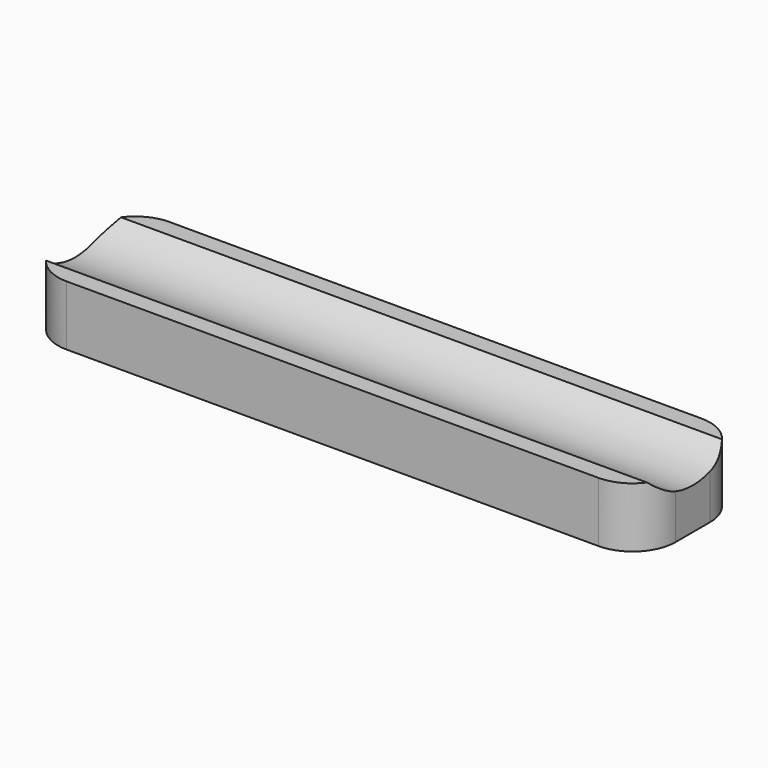
from build123d import *

# Parameters (mm, degrees)
F0_W      = 72
F0_H      = 15
F1_DEPTH  = 3.8
F3_DEPTH  = 72
F4_R      = 5
F5_W      = 36
F5_H      = 2
F6_DEPTH  = 1
F7_R      = 0.99999
F10_DEPTH = 4
F11_R     = 2
F12_R     = 1


# Not quite as in the source:
# - a fillet or chamfer is up to 0.001 mm smaller than in the source, because OpenCascade refuses the exact size
# - a pattern or mirror of a feature is missing from the dataset's text; its kind, count and spacing are read off the source's solid


with BuildPart() as f1:
    # F0 (on Top) → F1 (new body)
    with BuildSketch(Plane.XY):
        Rectangle(F0_W, F0_H)
    extrude(amount=F1_DEPTH)

    # F2 (on face) → F3 (join)
    with BuildSketch(Plane.YZ.offset(36)):
        with BuildLine():
            Line((7.5, 7), (5.4598534779, 7))
            ThreePointArc((5.4598534779, 7), (0, 4.8), (-5.4598534779, 7))
            Line((-5.4598534779, 7), (-7.5, 7))
            Line((-7.5, 7), (-7.5, 3.8))
            Line((-7.5, 3.8), (7.5, 3.8))
            Line((7.5, 3.8), (7.5, 7))
        make_face()
    extrude(amount=-F3_DEPTH)

    # F4
    f4_edges = [f1.edges().sort_by_distance(p)[0] for p in [
        (-36, -7.5, 3.5),
        (36, -7.5, 3.5),
        (36, 7.5, 3.5),
        (-36, 7.5, 3.5),
    ]]
    fillet(f4_edges, radius=F4_R)

    # F5 (on face) → F6 (cut)
    with BuildSketch(Plane(origin=(0, 0, 0), x_dir=(1, 0, 0), z_dir=(0, 0, -1))):
        Rectangle(F5_W, F5_H)
    extrude(amount=-F6_DEPTH, mode=Mode.SUBTRACT)

    # F7 (radius 1 in the source; OpenCascade refuses exactly that, so slightly less here)
    f7_edges = [f1.edges().sort_by_distance(p)[0] for p in [
        (0, -1, 1),
        (0, 1, 1),
    ]]
    fillet(f7_edges, radius=F7_R)

    # F9 (on offset) → F10 (cut)
    with BuildSketch(Plane.YZ.offset(16)):
        Polygon((-3.8, 0), (-1.8, 0), (-1.8, 1.8), (0, 1.8), (1.8, 1.8), (1.8, 0), (3.8, 0), (3.8, 3.8), (0, 3.8), (-3.8, 3.8), align=None)
    f10 = extrude(amount=-F10_DEPTH, mode=Mode.SUBTRACT)

    # F10_copies: F10 across plane
    add(f10.mirror(Plane(origin=(0, 0, 0), x_dir=(0, 0, -1), z_dir=(-1, 0, 0))), mode=Mode.SUBTRACT)

    # F11
    f11_edges = [f1.edges().sort_by_distance(p)[0] for p in [
        (14, -3.8, 3.8),
        (14, 3.8, 3.8),
        (-14, -3.8, 3.8),
        (-14, 3.8, 3.8),
    ]]
    fillet(f11_edges, radius=F11_R)

    # F12
    f12_edges = [f1.edges().sort_by_distance(p)[0] for p in [
        (14, -1.8, 1.8),
        (14, 1.8, 1.8),
        (-14, 1.8, 1.8),
        (-14, -1.8, 1.8),
    ]]
    fillet(f12_edges, radius=F12_R)


solid = f1.part
